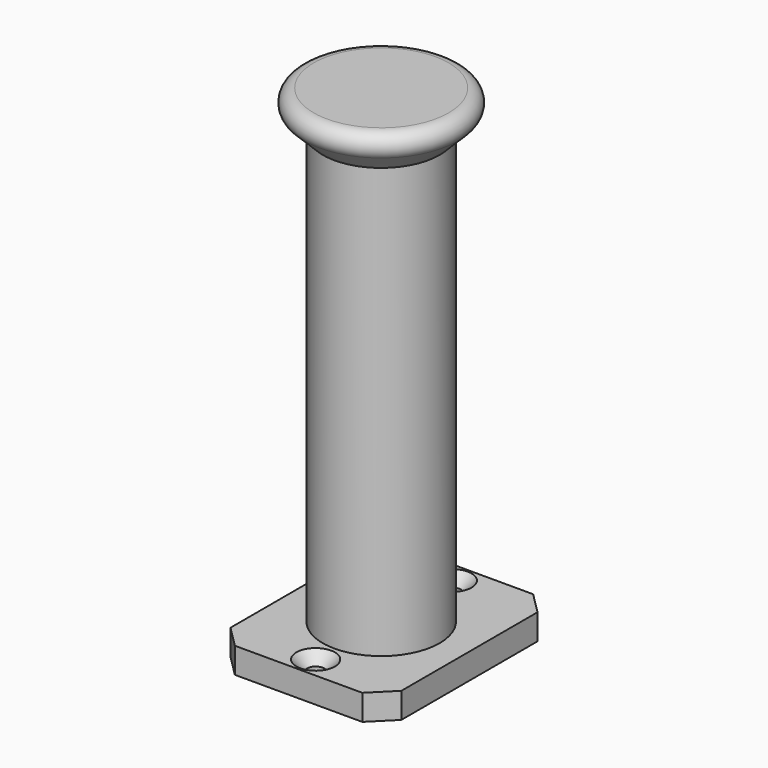
from build123d import *

# Parameters (mm, degrees)
F0_W        = 40
F0_H        = 50
F0_R        = 2
F1_DEPTH    = 6
F2_R        = 13.6797776514
F3_DEPTH    = 100
F4_R        = 23.0640267833
F5_DEPTH    = 10
F6_S5_R     = 13.6797776514
F6_T6_DEPTH = 34
F7_R        = 3
F8_SIZE     = 5.08
F9_SIZE     = 2.5


# Not quite as in the source:
# - a fillet or chamfer that OpenCascade refuses, or shapes differently, is made with other operations: its cross-section is extruded or revolved along the edge and cut away or added


with BuildPart() as f1:
    # F0 (on Top) → F1 (new body)
    with BuildSketch(Plane.XY):
        with Locations((20, 25)):
            Rectangle(F0_W, F0_H)
        with Locations((20, 5)):
            Circle(F0_R, mode=Mode.SUBTRACT)
        with Locations((20, 45)):
            Circle(F0_R, mode=Mode.SUBTRACT)
    extrude(amount=F1_DEPTH)

    # F2 (on face) → F3 (join)
    with BuildSketch(Plane.XY.offset(6)):
        with Locations((20, 24.1802949458)):
            Circle(F2_R)
    extrude(amount=F3_DEPTH)

    # F4 (on face) → F5 (join)
    with BuildSketch(Plane.XY.offset(106)):
        with Locations((20, 24.1802949458)):
            Circle(F4_R)
    extrude(amount=F5_DEPTH)

    # F6: chamfer of 10 on 1 edges, made by hand


with BuildPart() as f6_tool2:
    # F6_s3 → F6_t4 (revolve)
    with BuildSketch(Plane.XZ.offset(-24.1802949458)):
        Polygon((43.0640267833, 116), (33.0640267833, 106), (43.0640267833, 106), align=None)
    revolve(axis=Axis((20, 24.1802949458, 106), (0, 0, 1)))

    # F6_s5 → F6_t6 (cut, symmetric)
    with BuildSketch(Plane.XY.offset(111)):
        with Locations((20, 24.1802949458)):
            Circle(F6_S5_R)
    extrude(amount=F6_T6_DEPTH, both=True, mode=Mode.SUBTRACT)


with BuildPart() as f1_1:
    add(f1.part)

    # F6_t1: cut F6_tool2
    add(f6_tool2.part, mode=Mode.SUBTRACT)

    # F7
    f7_edges = [f1_1.edges().sort_by_distance(p)[0] for p in [
        (-3.064027, 24.180295, 116),
    ]]
    fillet(f7_edges, radius=F7_R)

    # F8
    f8_edges = [f1_1.edges().sort_by_distance(p)[0] for p in [
        (40, 0, 3),
        (40, 50, 3),
        (0, 50, 3),
        (0, 0, 3),
    ]]
    chamfer(f8_edges, length=F8_SIZE)

    # F9
    f9_edges = [f1_1.edges().sort_by_distance(p)[0] for p in [
        (18, 5, 6),
        (18, 45, 6),
    ]]
    chamfer(f9_edges, length=F9_SIZE)


solid = f1_1.part
